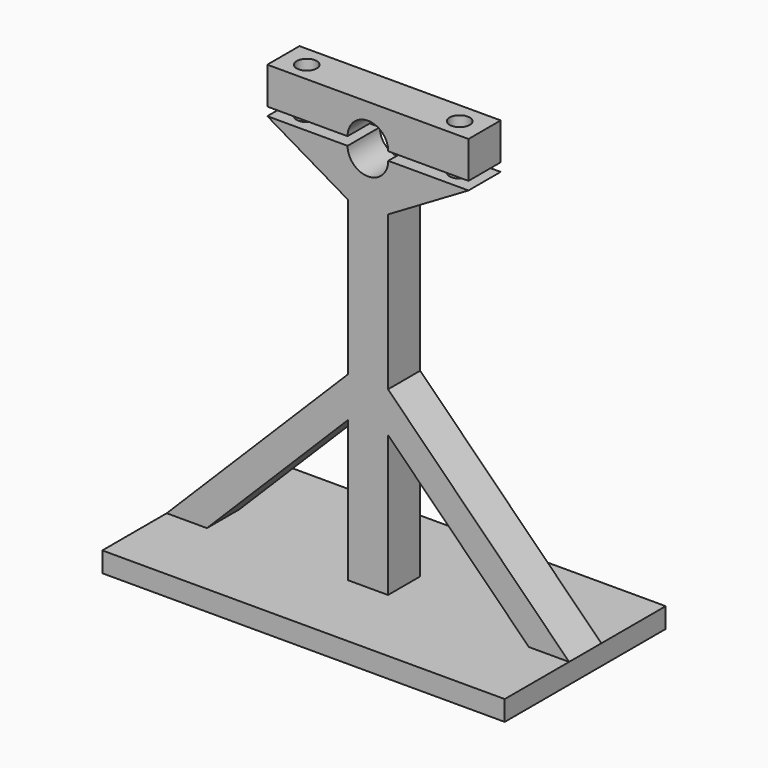
from build123d import *

# Parameters (mm, degrees)
F1_DEPTH = 10
F3_R     = 2.5
F4_DEPTH = 25
F5_W     = 100
F5_H     = 20
F6_DEPTH = 5


# Not quite as in the source:
# - a feature names something its author has since deleted; it is built from what else it names


with BuildPart() as f1:
    # F0 (on Front) → F1 (new body)
    with BuildSketch(Plane.XZ):
        with BuildLine():
            Line((-5.05, 50), (-25, 50))
            Line((-25, 50), (-5, 38.2643528283))
            Line((-5, 38.2643528283), (-5, 0))
            Line((-5, 0), (-50, -45))
            Line((-50, -45), (-50, -50))
            Line((-50, -50), (50, -50))
            Line((50, -50), (50, -45))
            Line((50, -45), (5, 0))
            Line((5, 0), (5, 38.2643528283))
            Line((5, 38.2643528283), (25, 50))
            Line((25, 50), (5.05, 50))
            ThreePointArc((5.05, 50), (0, 44.95), (-5.05, 50))
        make_face()
        Polygon((-5, -45), (-40, -45), (-5, -10), align=None, mode=Mode.SUBTRACT)
        Polygon((5, -10), (40, -45), (5, -45), align=None, mode=Mode.SUBTRACT)
    extrude(amount=F1_DEPTH)


with BuildPart() as f1b:
    # F0 (on Front) → F1, piece 2 (new body)
    with BuildSketch(Plane.XZ):
        with BuildLine():
            Line((5.05, 52.1000094712), (25, 52.1000094712))
            Line((25, 52.1000094712), (25, 61.2651444972))
            Line((25, 61.2651444972), (-25, 61.2651444972))
            Line((-25, 61.2651444972), (-25, 52.1000094712))
            Line((-25, 52.1000094712), (-5.05, 52.1000094712))
            ThreePointArc((-5.05, 52.1000094712), (0, 57.1500094712), (5.05, 52.1000094712))
        make_face()
    extrude(amount=F1_DEPTH)


with BuildPart() as f4_tool:
    # F3 (on offset) → F4 (new body)
    with BuildSketch(Plane.XY.offset(61.5)):
        with Locations((-19, -5.2368245088)):
            Circle(F3_R)
        with Locations((19, -5.2368245088)):
            Circle(F3_R)
    extrude(amount=-F4_DEPTH)


with BuildPart() as f1_1:
    add(f1.part)

    # F4: cut by f4_tool
    add(f4_tool.part, mode=Mode.SUBTRACT)

    # F5 (on face) → F6 (join)
    with BuildSketch(Plane(origin=(0, 0, -50), x_dir=(1, 0, 0), z_dir=(0, 0, -1))):
        with Locations((0, -10)):
            Rectangle(F5_W, F5_H)
        with Locations((0, 20)):
            Rectangle(F5_W, F5_H)
    extrude(amount=-F6_DEPTH)


with BuildPart() as f1b_1:
    add(f1b.part)

    # F4: cut by f4_tool
    add(f4_tool.part, mode=Mode.SUBTRACT)


solid = Compound([f1_1.part, f1b_1.part])
